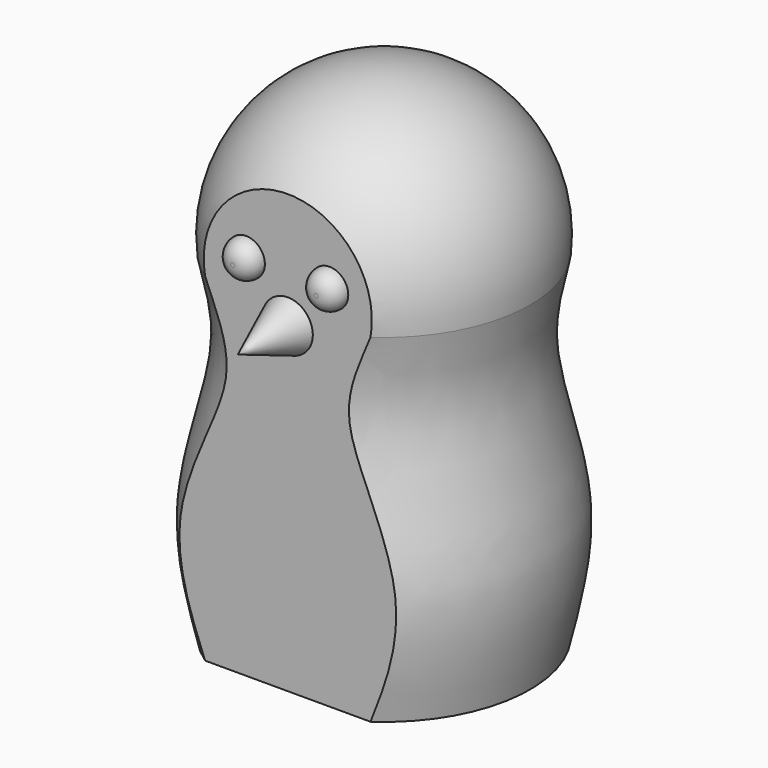
from build123d import *

# Parameters (mm, degrees)
F3_DEPTH  = 177.8
F4_R      = 7.62
F5_DEPTH  = 19.05
F6_SIZE2  = 18.860161823
F6_SIZE   = 7.62
F4_R_2    = 5.715
F7_DEPTH  = 5.08
F8_R      = 5.07999
F9_R      = 6.35
F10_DEPTH = 50.8
F11_SCALE = 0.85684223


# Not quite as in the source:
# - a fillet or chamfer is up to 0.001 mm smaller than in the source, because OpenCascade refuses the exact size


with BuildPart() as f1:
    # F0 (on Front) → F1 (revolve)
    with BuildSketch(Plane.XZ):
        with BuildLine():
            Line((-38.2711647941, 0), (0, 0))
            Line((0, 0), (0, 146.0500033258))
            Line((0, 146.0500033258), (0, 152.4))
            ThreePointArc((0, 152.4), (-33.2006597867, 137.6319951518), (-44.4655865431, 103.0852268133))
            add(Edge.make_bspline(
                [(-44.4655865431, 0), (-47.1114422222, 11.762074058), (-53.3469479224, 35.8297600734), (-37.8272166921, 76.0482431769), (-42.543614325, 94.8604386904), (-44.4655865431, 103.0852268133)],
                knots=[0, 0, 0, 0, 0.3424224234, 0.7066775859, 1, 1, 1, 1], degree=3))
            Line((-44.4655865431, 0), (-38.2711647941, 0))
        make_face()
    revolve(axis=Axis((0, 0, 76.2), (0, 0, 1)))

    # F2 (on Top) → F3 (cut)
    with BuildSketch(Plane.XY):
        Polygon((25.6092443837, -36.641700535), (-25.1907556163, -36.641700535), (-46.7807556163, -36.641700535), (-46.7807556163, -67.121700535), (42.1192443837, -67.121700535), (42.1192443837, -36.641700535), align=None)
    extrude(amount=F3_DEPTH, mode=Mode.SUBTRACT)

    # F4 (on face) → F5 (join)
    with BuildSketch(Plane.XZ.offset(36.641700535)):
        with Locations((0, 97.9992443837)):
            Circle(F4_R)
    extrude(amount=F5_DEPTH)

    # F6
    f6_edges = [f1.edges().sort_by_distance(p)[0] for p in [
        (-7.62, -55.691701, 97.999244),
    ]]
    f6_side = f1.faces().sort_by_distance((0, -55.691701, 97.999244))[0]
    chamfer(f6_edges, length=F6_SIZE, length2=F6_SIZE2, reference=f6_side)

    # F4 (on face) → F7 (join)
    with BuildSketch(Plane.XZ.offset(36.641700535)):
        with Locations((-12.7, 112.2232443837)):
            Circle(F4_R_2)
        with Locations((12.7, 112.2232443837)):
            Circle(F4_R_2)
    extrude(amount=F7_DEPTH)

    # F8 (radius 5.08 in the source; OpenCascade refuses exactly that, so slightly less here)
    f8_edges = [f1.edges().sort_by_distance(p)[0] for p in [
        (-18.415, -41.721701, 112.223244),
        (6.985, -41.721701, 112.223244),
    ]]
    fillet(f8_edges, radius=F8_R)

    # F9 (on face) → F10 (cut)
    with BuildSketch(Plane(origin=(0, 0, 0), x_dir=(1, 0, 0), z_dir=(0, 0, -1))):
        Circle(F9_R)
    extrude(amount=-F10_DEPTH, mode=Mode.SUBTRACT)


with BuildPart() as f1_1:
    # F11: moved
    add(f1.part.scale(F11_SCALE))


solid = f1_1.part
